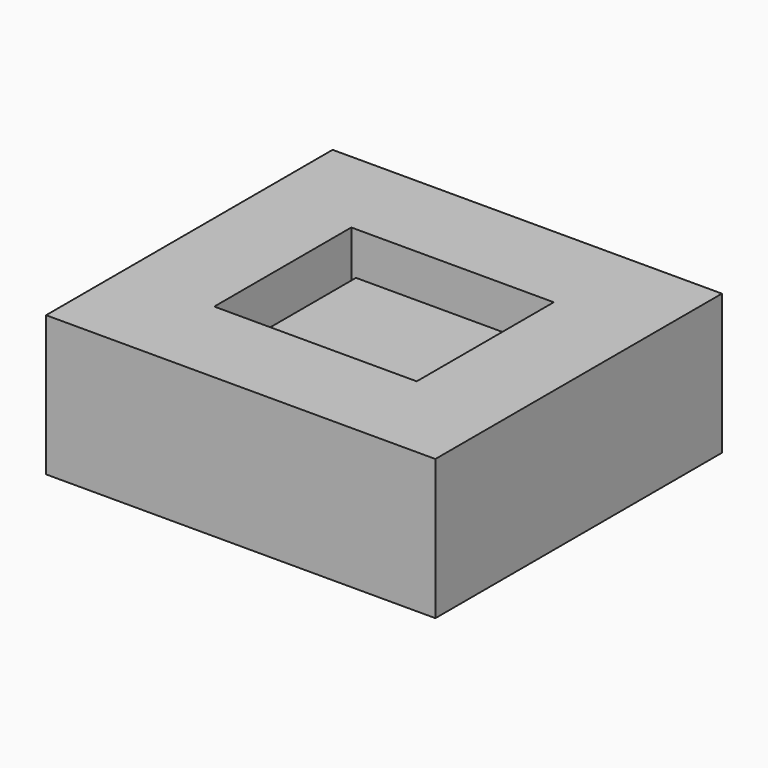
from build123d import *

# Parameters (mm, degrees)
F2_W          = 20
F2_H          = 16
F3_DEPTH      = 11.5
F4_W          = 50
F4_H          = 46
F4_W_2        = 26
F4_H_2        = 22
F5_DEPTH      = 15
F5_DEPTH_BACK = 3
F6_DEPTH      = 25


with BuildPart() as f1:
    # F0 (on Front) → F1 (revolve)
    with BuildSketch(Plane.XZ):
        Polygon((-10.6553274116, -3.7553449435), (-10, -3), (-13.7545470851, 0.3020260729), (-14.4149372893, -0.4488662767), align=None)
    revolve(axis=Axis((0, 0, 14.246087247), (0, 0, 1)))


with BuildPart() as f3:
    # F2 (on Top) → F3 (new body)
    with BuildSketch(Plane.XY):
        with Locations((5.5, 0)):
            Rectangle(F2_W, F2_H)
    extrude(amount=F3_DEPTH)


with BuildPart() as f5:
    # F4 (on Top) → F5 (new body, two sides)
    with BuildSketch(Plane.XY) as f5_sk:
        with Locations((5.5, 0)):
            Rectangle(F4_W, F4_H)
        with Locations((5.5, 0)):
            Rectangle(F4_W_2, F4_H_2, mode=Mode.SUBTRACT)
        with Locations((5.5, 0)):
            Rectangle(F4_W_2, F4_H_2)
    extrude(amount=F5_DEPTH)
    extrude(f5_sk.sketch, amount=-F5_DEPTH_BACK)

    # F4 (on Top) → F6 (cut)
    with BuildSketch(Plane.XY):
        with Locations((5.5, 0)):
            Rectangle(F4_W_2, F4_H_2)
    extrude(amount=F6_DEPTH, mode=Mode.SUBTRACT)


solid = Compound([f1.part, f3.part, f5.part])
